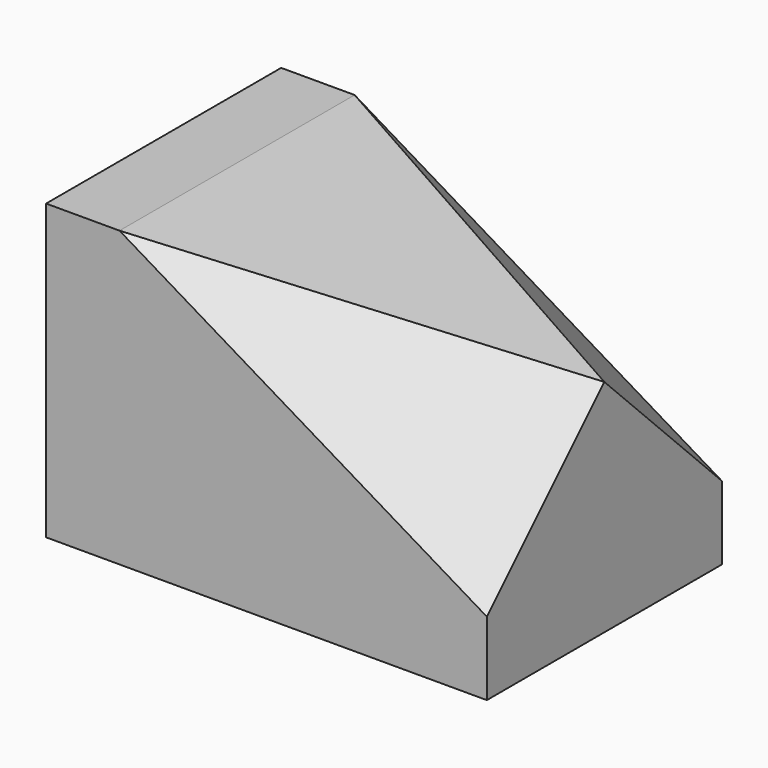
from build123d import *

# Parameters (mm, degrees)
F0_W      = 60
F0_H      = 40
F1_DEPTH  = 40
F2_SIZE2  = 10
F2_SIZE   = 50
F7_DEPTH  = 19.5293366471
F11_DEPTH = 19.5293366471


with BuildPart() as f1:
    # F0 (on Top) → F1 (new body)
    with BuildSketch(Plane.XY):
        with Locations((30, 20)):
            Rectangle(F0_W, F0_H)
    extrude(amount=F1_DEPTH)

    # F2
    f2_edges = [f1.edges().sort_by_distance(p)[0] for p in [
        (60, 20, 40),
    ]]
    f2_side = f1.faces().sort_by_distance((30, 20, 40))[0]
    chamfer(f2_edges, length=F2_SIZE, length2=F2_SIZE2, reference=f2_side)

    # F6 (on face) → F7 (cut, through all)
    with BuildSketch(Plane(origin=(11.6949152542, -19.4915254237, 19.4915254237), x_dir=(0.9205746179, 0.2761723854, -0.2761723854), z_dir=(0.3905667329, -0.6509445549, 0.6509445549))):
        Polygon((52.4727532202, 35.3553390593), (-1.8411492358, 28.2842712475), (52.4727532202, 7.0710678119), align=None)
    extrude(amount=F7_DEPTH, mode=Mode.SUBTRACT)

    # F10 (on face) → F11 (cut, through all)
    with BuildSketch(Plane(origin=(21.8644067797, 36.4406779661, 36.4406779661), x_dir=(0.9205746179, -0.2761723854, -0.2761723854), z_dir=(-0.3905667329, -0.6509445549, -0.6509445549))):
        Polygon((41.4258578054, 7.0710678119), (-12.8880446506, 0), (41.4258578054, -21.2132034356), align=None)
    extrude(amount=-F11_DEPTH, mode=Mode.SUBTRACT)


solid = f1.part
